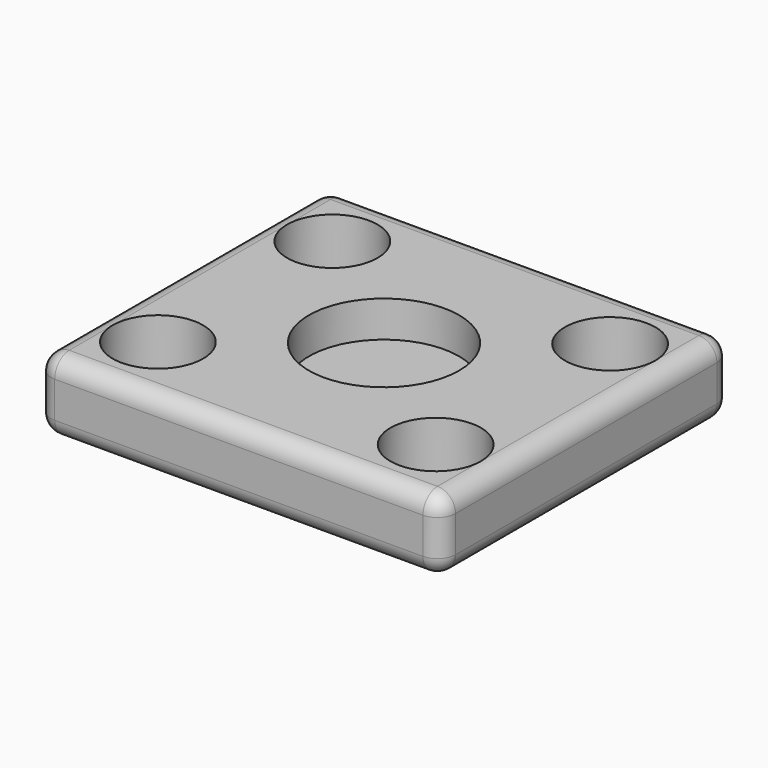
from build123d import *

# Parameters (mm, degrees)
F0_W     = 44.7
F0_H     = 40.1
F0_R     = 5
F0_R_2   = 8.3
F1_DEPTH = 8
F2_DEPTH = 4
F0_R_3   = 4
F3_DEPTH = 1
F4_R     = 1.99999


# Not quite as in the source:
# - a fillet or chamfer is up to 0.001 mm smaller than in the source, because OpenCascade refuses the exact size


with BuildPart() as f1:
    # F0 (on Top) → F1 (new body)
    with BuildSketch(Plane.XY):
        Rectangle(F0_W, F0_H)
        with Locations((-15.35, -12.05)):
            Circle(F0_R, mode=Mode.SUBTRACT)
        with Locations((15.35, -12.05)):
            Circle(F0_R, mode=Mode.SUBTRACT)
        Circle(F0_R_2, mode=Mode.SUBTRACT)
        with Locations((-15.35, 12.05)):
            Circle(F0_R, mode=Mode.SUBTRACT)
        with Locations((15.35, 12.05)):
            Circle(F0_R, mode=Mode.SUBTRACT)
    extrude(amount=F1_DEPTH)

    # F0 (on Top) → F2 (join)
    with BuildSketch(Plane.XY):
        Circle(F0_R_2)
    extrude(amount=F2_DEPTH)

    # F0 (on Top) → F3 (join)
    with BuildSketch(Plane.XY):
        with Locations((15.35, 12.05)):
            Circle(F0_R)
        with Locations((15.35, 12.05)):
            Circle(F0_R_3, mode=Mode.SUBTRACT)
        with Locations((15.35, -12.05)):
            Circle(F0_R)
        with Locations((15.35, -12.05)):
            Circle(F0_R_3, mode=Mode.SUBTRACT)
        with Locations((-15.35, -12.05)):
            Circle(F0_R)
        with Locations((-15.35, -12.05)):
            Circle(F0_R_3, mode=Mode.SUBTRACT)
        with Locations((-15.35, 12.05)):
            Circle(F0_R)
        with Locations((-15.35, 12.05)):
            Circle(F0_R_3, mode=Mode.SUBTRACT)
    extrude(amount=F3_DEPTH)

    # F4 (radius 2 in the source; OpenCascade refuses exactly that, so slightly less here)
    f4_edges = [f1.edges().sort_by_distance(p)[0] for p in [
        (0, 20.05, 8),
        (-22.35, 0, 8),
        (0, -20.05, 8),
        (22.35, 0, 8),
        (0, -20.05, 0),
        (-22.35, 0, 0),
        (-22.35, -20.05, 4),
        (22.35, -20.05, 4),
        (22.35, 0, 0),
        (22.35, 20.05, 4),
        (0, 20.05, 0),
        (-22.35, 20.05, 4),
    ]]
    fillet(f4_edges, radius=F4_R)


solid = f1.part
